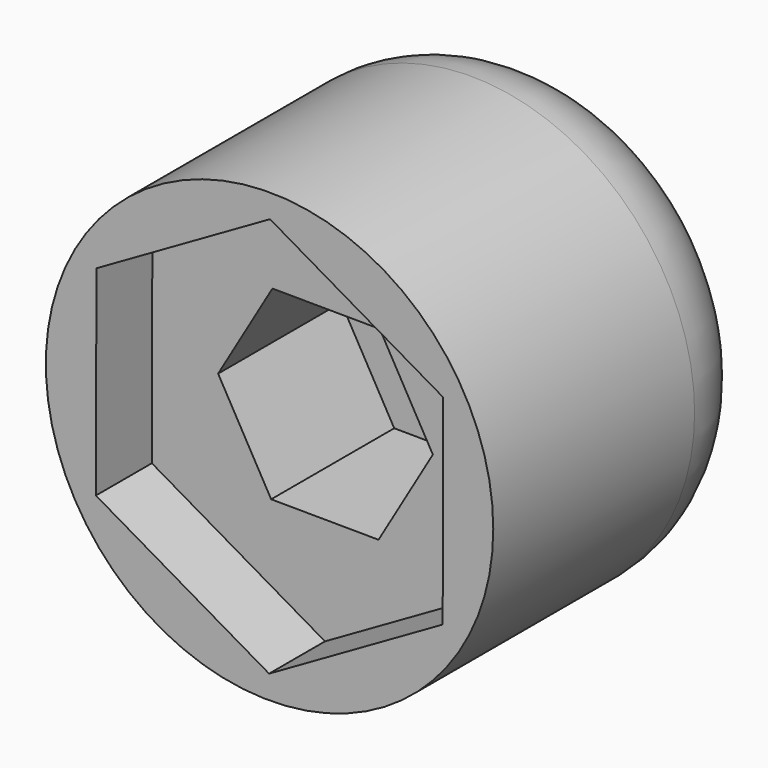
from build123d import *

# Parameters (mm, degrees)
F0_R     = 16
F1_DEPTH = 21
F0_R_2   = 9
F2_DEPTH = 16
F3_R     = 16
F4_DEPTH = 4
F5_DEPTH = 16
F6_R     = 7
F0_R_3   = 4.2
F7_DEPTH = 5


with BuildPart() as f1:
    # F0 (on Front) → F1 (new body)
    with BuildSketch(Plane.XZ):
        Circle(F0_R)
        Polygon((-12.417059955, -7.1295129852), (-12.3828693393, 7.1887328687), (0.0341906157, 14.318245854), (12.417059955, 7.1295129852), (12.3828693393, -7.1887328687), (-0.0341906157, -14.318245854), align=None, mode=Mode.SUBTRACT)
    extrude(amount=F1_DEPTH)



with BuildPart() as f2:
    # F0 (on Front) → F2 (new body)
    with BuildSketch(Plane.XZ):
        Circle(F0_R_2)
        Polygon((-3.8840263382, -6.6240223986), (-7.6785848415, 0.0516542785), (-3.7945585034, 6.6756766771), (3.8840263382, 6.6240223986), (7.6785848415, -0.0516542785), (3.7945585034, -6.6756766771), align=None, mode=Mode.SUBTRACT)
    extrude(amount=F2_DEPTH)


with BuildPart() as f1_1:
    add(f1.part)

    add(f2.part)  # F4 merges F2
    # F3 (on Front) → F4 (join)
    with BuildSketch(Plane.XZ):
        Circle(F3_R)
    extrude(amount=-F4_DEPTH)

    # F0 (on Front) → F5 (join)
    with BuildSketch(Plane.XZ):
        Polygon((0.0341906157, 14.318245854), (-12.3828693393, 7.1887328687), (-12.417059955, -7.1295129852), (-0.0341906157, -14.318245854), (12.3828693393, -7.1887328687), (12.417059955, 7.1295129852), align=None)
        Circle(F0_R_2, mode=Mode.SUBTRACT)
    extrude(amount=F5_DEPTH)

    # F6
    f6_edges = [f1_1.edges().sort_by_distance(p)[0] for p in [
        (-16, 4, 0),
    ]]
    fillet(f6_edges, radius=F6_R)

    # F0 (on Front) → F7 (join)
    with BuildSketch(Plane.XZ):
        Polygon((-3.7945585034, 6.6756766771), (-7.6785848415, 0.0516542785), (-3.8840263382, -6.6240223986), (3.7945585034, -6.6756766771), (7.6785848415, -0.0516542785), (3.8840263382, 6.6240223986), align=None)
        Circle(F0_R_3, mode=Mode.SUBTRACT)
    extrude(amount=F7_DEPTH)


solid = f1_1.part
